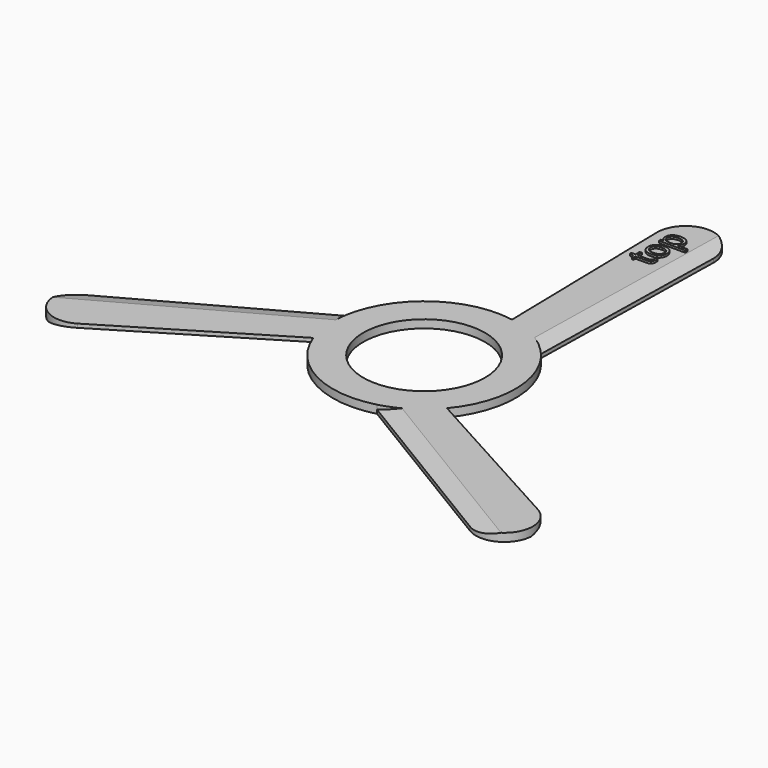
from build123d import *

# Parameters (mm, degrees)
F0_R         = 30
F1_DEPTH     = 4
F2_T4_DEPTH  = 132.9709225207
F2_S5_R      = 45
F2_T6_DEPTH  = 68
F2_T10_DEPTH = 132.9709225207
F2_S11_R     = 45
F2_T12_DEPTH = 71
F2_T16_DEPTH = 132.9709225207
F2_S17_R     = 45
F2_T18_DEPTH = 72
F2_T22_DEPTH = 145.5118337832
F2_S23_R     = 45
F2_T24_DEPTH = 78
F2_T28_DEPTH = 145.5118337832
F2_S29_R     = 45
F2_T30_DEPTH = 75
F2_T34_DEPTH = 145.5118337832
F2_S35_R     = 45
F2_T36_DEPTH = 78
F3_TEXT_SIZE = 16.6666666667
F4_DEPTH     = 1
F5_TEXT_SIZE = 16.6666666667
F6_DEPTH     = 1


# Not quite as in the source:
# - a fillet or chamfer that OpenCascade refuses, or shapes differently, is made with other operations: its cross-section is extruded or revolved along the edge and cut away or added
# - Text() gives the source's letters only with a copy of the font that has no kerning and outlines rounded to 1/6400 em; it was checked with that copy


with BuildPart() as f1:
    # F0 (on Top) → F1 (new body)
    with BuildSketch(Plane.XY):
        with BuildLine():
            Line((114.5286501005, -73.0513501957), (34.4344606986, -28.9701210974))
            ThreePointArc((34.4344606986, -28.9701210974), (44.9599943305, 1.8970792813), (31.8716304717, 31.7678952887))
            Line((31.8716304717, 31.7678952887), (34, 135.710395546))
            ThreePointArc((34, 135.710395546), (20, 150), (6, 135.710395546))
            Line((6, 135.710395546), (7.8716304717, 44.3061782793))
            ThreePointArc((7.8716304717, 44.3061782793), (-24.1229160158, 37.9879576036), (-43.4476195806, 11.7176940042))
            Line((-43.4476195806, 11.7176940042), (-134.5286501005, -38.4103340443))
            ThreePointArc((-134.5286501005, -38.4103340443), (-139.9038105677, -57.6794919243), (-120.5286501005, -62.6590453503))
            Line((-120.5286501005, -62.6590453503), (-42.3060911703, -15.3360571819))
            ThreePointArc((-42.3060911703, -15.3360571819), (-20.8370783147, -39.8850368849), (11.5759891089, -43.4855892929))
            Line((11.5759891089, -43.4855892929), (100.5286501005, -97.3000615017))
            ThreePointArc((100.5286501005, -97.3000615017), (119.9038105677, -92.3205080757), (114.5286501005, -73.0513501957))
        make_face()
        Circle(F0_R, mode=Mode.SUBTRACT)
    extrude(amount=F1_DEPTH)

    # F2: chamfer of 8 x 2.1435935394 on 6 edges, made by hand


with BuildPart() as f2_tool2:
    # F2_s3 → F2_t4 (new body)
    with BuildSketch(Plane(origin=(-3.2004659642, 156.3001301632, 0), x_dir=(0, 0, 1), z_dir=(0.0204721213, -0.9997904242, 0))):
        Polygon((2.1435935394, -8.7770222242), (0, -16.7770222242), (0, -8.7770222242), align=None)
    extrude(amount=F2_T4_DEPTH)

    # F2_s5 → F2_t6 (cut, symmetric)
    with BuildSketch(Plane.XY.offset(1.1)):
        Circle(F2_S5_R)
    extrude(amount=F2_T6_DEPTH, both=True, mode=Mode.SUBTRACT)


with BuildPart() as f1_1:
    add(f1.part)

    # F2_t1: cut F2_tool2
    add(f2_tool2.part, mode=Mode.SUBTRACT)


with BuildPart() as f2_tool8:
    # F2_s9 → F2_t10 (new body)
    with BuildSketch(Plane(origin=(136.9601163183, -75.3783802527, 0), x_dir=(0, 0, 1), z_dir=(-0.8760799664, 0.482165835, 0))):
        Polygon((2.1435935394, -8.7770222242), (0, -16.7770222242), (0, -8.7770222242), align=None)
    extrude(amount=F2_T10_DEPTH)

    # F2_s11 → F2_t12 (cut, symmetric)
    with BuildSketch(Plane.XY.offset(1.1)):
        Circle(F2_S11_R)
    extrude(amount=F2_T12_DEPTH, both=True, mode=Mode.SUBTRACT)


with BuildPart() as f1_2:
    add(f1_1.part)

    # F2_t7: cut F2_tool8
    add(f2_tool8.part, mode=Mode.SUBTRACT)


with BuildPart() as f2_tool14:
    # F2_s15 → F2_t16 (new body)
    with BuildSketch(Plane(origin=(-133.7596503541, -80.9217499106, 0), x_dir=(0, 0, 1), z_dir=(0.8556078451, 0.5176245892, 0))):
        Polygon((2.1435935394, -8.7770222242), (0, -16.7770222242), (0, -8.7770222242), align=None)
    extrude(amount=F2_T16_DEPTH)

    # F2_s17 → F2_t18 (cut, symmetric)
    with BuildSketch(Plane.XY.offset(1.1)):
        Circle(F2_S17_R)
    extrude(amount=F2_T18_DEPTH, both=True, mode=Mode.SUBTRACT)


with BuildPart() as f1_3:
    add(f1_2.part)

    # F2_t13: cut F2_tool14
    add(f2_tool14.part, mode=Mode.SUBTRACT)


with BuildPart() as f2_tool20:
    # F2_s21 → F2_t22 (new body)
    with BuildSketch(Plane(origin=(9.9592281126, -6.0251216603, 0), x_dir=(0, 0, 1), z_dir=(0.8556078451, -0.5176245892, 0))):
        Polygon((1.8564064606, 31.2145947423), (4, 23.2145947423), (4, 31.2145947423), align=None)
    extrude(amount=F2_T22_DEPTH)

    # F2_s23 → F2_t24 (cut, symmetric)
    with BuildSketch(Plane.XY.offset(2.9)):
        Circle(F2_S23_R)
    extrude(amount=F2_T24_DEPTH, both=True, mode=Mode.SUBTRACT)


with BuildPart() as f1_4:
    add(f1_3.part)

    # F2_t19: cut F2_tool20
    add(f2_tool20.part, mode=Mode.SUBTRACT)


with BuildPart() as f2_tool26:
    # F2_s27 → F2_t28 (new body)
    with BuildSketch(Plane(origin=(0.2382943625, 11.6375053778, 0), x_dir=(0, 0, 1), z_dir=(0.0204721213, 0.9997904242, 0))):
        Polygon((1.8564064606, 31.2145947423), (4, 23.2145947423), (4, 31.2145947423), align=None)
    extrude(amount=F2_T28_DEPTH)

    # F2_s29 → F2_t30 (cut, symmetric)
    with BuildSketch(Plane.XY.offset(2.9)):
        Circle(F2_S29_R)
    extrude(amount=F2_T30_DEPTH, both=True, mode=Mode.SUBTRACT)


with BuildPart() as f1_5:
    add(f1_4.part)

    # F2_t25: cut F2_tool26
    add(f2_tool26.part, mode=Mode.SUBTRACT)


with BuildPart() as f2_tool32:
    # F2_s33 → F2_t34 (new body)
    with BuildSketch(Plane(origin=(-10.197522475, -5.6123837174, 0), x_dir=(0, 0, 1), z_dir=(-0.8760799664, -0.482165835, 0))):
        Polygon((1.8564064606, 31.2145947423), (4, 23.2145947423), (4, 31.2145947423), align=None)
    extrude(amount=F2_T34_DEPTH)

    # F2_s35 → F2_t36 (cut, symmetric)
    with BuildSketch(Plane.XY.offset(2.9)):
        Circle(F2_S35_R)
    extrude(amount=F2_T36_DEPTH, both=True, mode=Mode.SUBTRACT)


with BuildPart() as f1_6:
    add(f1_5.part)

    # F2_t31: cut F2_tool32
    add(f2_tool32.part, mode=Mode.SUBTRACT)

    # F3 (on face) → F4 (join)
    with BuildSketch(Plane.XY.offset(4)):
        with Locations(Location((21.0995366616, 112.0487577831), (0, 0, 90))):
            Text('top', F3_TEXT_SIZE, font='Open Sans', text_align=(TextAlign.LEFT, TextAlign.BOTTOM))
    extrude(amount=F4_DEPTH)

    # F5 (on face) → F6 (join)
    with BuildSketch(Plane(origin=(0, 0, 0), x_dir=(1, 0, 0), z_dir=(0, 0, -1))):
        with Locations(Location((17.3466707954, -79.3666126603), (0, 0, -90))):
            Text('bottom', F5_TEXT_SIZE, font='Open Sans', text_align=(TextAlign.LEFT, TextAlign.BOTTOM))
    extrude(amount=F6_DEPTH)


solid = f1_6.part
